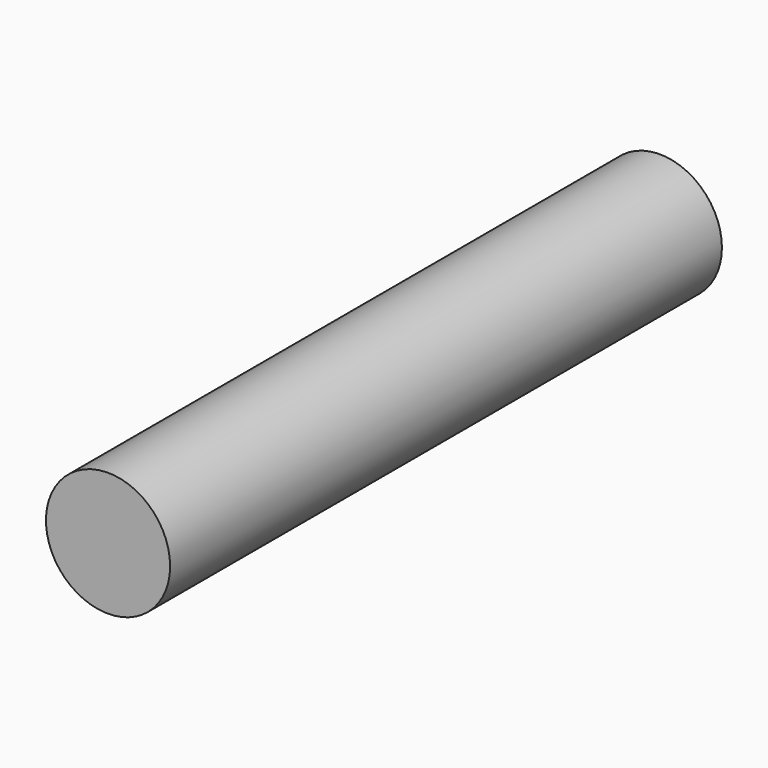
from build123d import *

# Parameters (mm, degrees)
F0_R     = 9
F1_DEPTH = 100


# Not quite as in the source:
# - a feature of the source that left no trace in its solid (it failed there, or was rolled back) is left out


with BuildPart() as f1:
    # F0 (on Front) → F1 (new body)
    with BuildSketch(Plane.XZ):
        Circle(F0_R)
    extrude(amount=F1_DEPTH)


solid = f1.part
